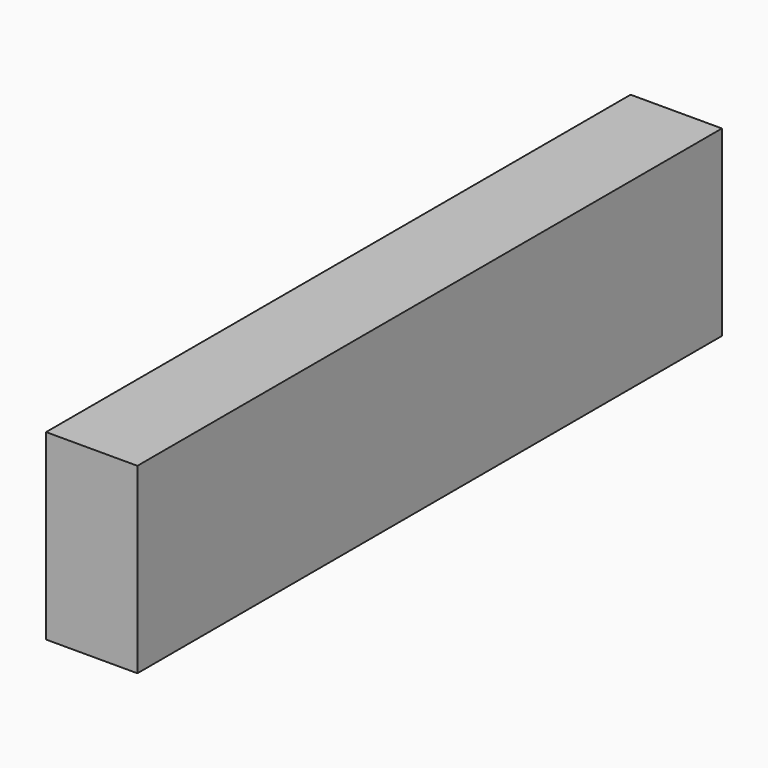
from build123d import *

# Parameters (mm, degrees)
F0_W     = 320
F0_H     = 80
F1_DEPTH = 20
F2_ANGLE = 90
F3_ANGLE = 90


with BuildPart() as f1:
    # F0 (on Top) → F1 (new body, symmetric)
    with BuildSketch(Plane.XY):
        Rectangle(F0_W, F0_H)
    extrude(amount=F1_DEPTH, both=True)


with BuildPart() as f1_1:
    # F2: moved
    add(f1.part.rotate(Axis((0, -40, -20), (1, 0, 0)), F2_ANGLE))


with BuildPart() as f1_2:
    # F3: moved
    add(f1_1.part.rotate(Axis((160, -40, 20), (0, 0, -1)), F3_ANGLE))


solid = f1_2.part
